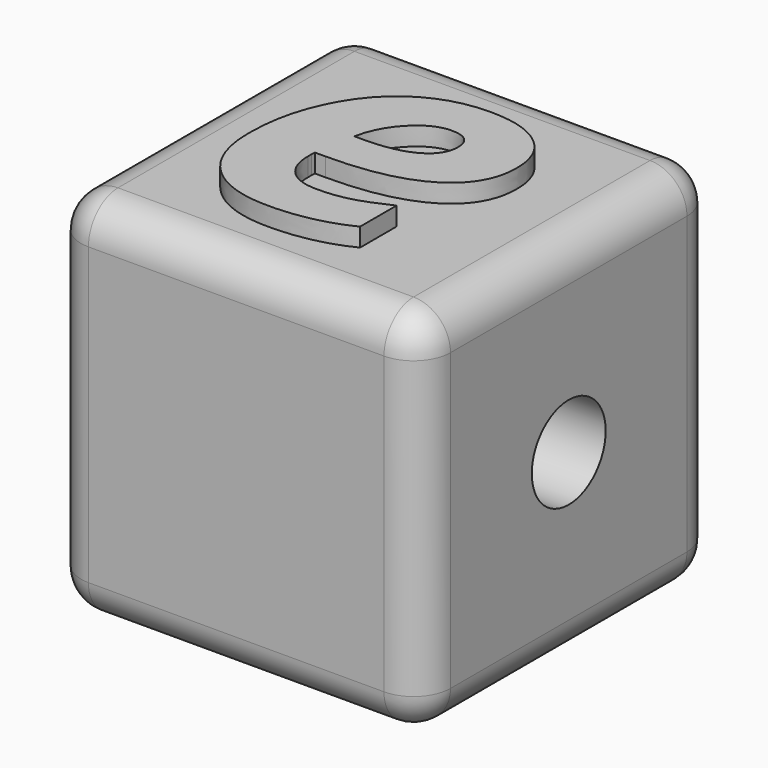
from build123d import *

# Parameters (mm, degrees)
F0_W         = 10
F0_H         = 10
F1_DEPTH     = 10
F2_R         = 1
F3_TEXT_SIZE = 11.1111111111
F4_DEPTH     = 0.5
F5_R         = 1.25
F6_DEPTH     = 25


# Not quite as in the source:
# - Text() gives the source's letters only with a copy of the font that has no kerning and outlines rounded to 1/6400 em; it was checked with that copy


with BuildPart() as f1:
    # F0 (on Top) → F1 (new body)
    with BuildSketch(Plane.XY):
        Rectangle(F0_W, F0_H)
    extrude(amount=F1_DEPTH)

    # F2
    f2_edges = [f1.edges().sort_by_distance(p)[0] for p in [
        (-5, 0, 0),
        (0, -5, 0),
        (5, 0, 0),
        (0, 5, 0),
        (-5, -5, 5),
        (5, -5, 5),
        (0, -5, 10),
        (5, 0, 10),
        (-5, 0, 10),
        (0, 5, 10),
        (5, 5, 5),
        (-5, 5, 5),
    ]]
    fillet(f2_edges, radius=F2_R)

    # F3 (on face) → F4 (join)
    with BuildSketch(Plane.XY.offset(10)):
        with Locations((-3.2974367924, -3.2974367924)):
            Text('e', F3_TEXT_SIZE, font='Open Sans', font_style=FontStyle.BOLDITALIC, text_align=(TextAlign.LEFT, TextAlign.BOTTOM))
    extrude(amount=F4_DEPTH)

    # F5 (on face) → F6 (cut)
    with BuildSketch(Plane.YZ.offset(5)):
        with Locations((0, 5)):
            Circle(F5_R)
    extrude(amount=-F6_DEPTH, mode=Mode.SUBTRACT)


solid = f1.part
